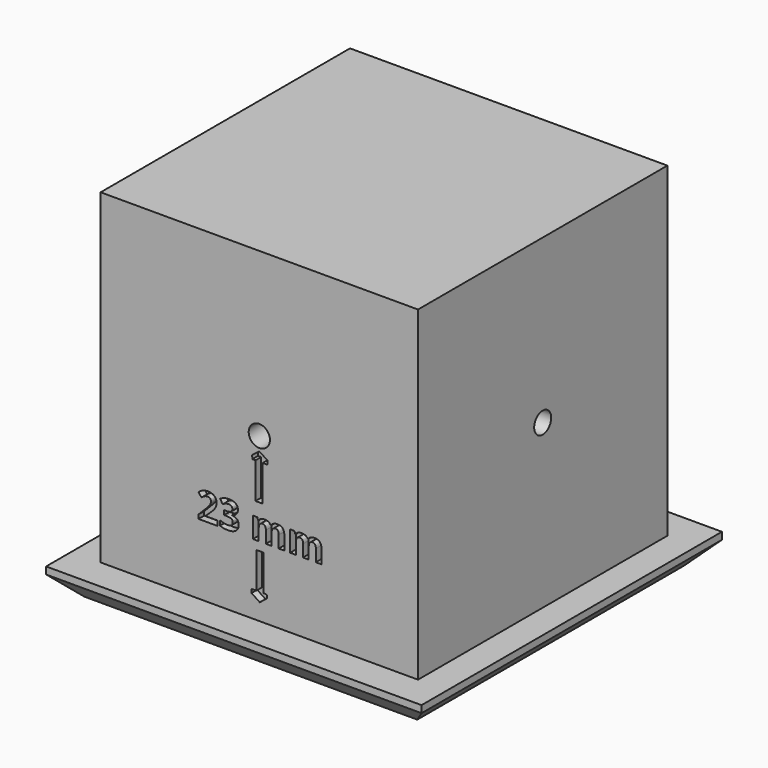
from build123d import *

# Parameters (mm, degrees)
F0_W          = 44.8
F0_H          = 44
F0_W_2        = 37.5
F0_H_2        = 37.5
F1_DEPTH      = 50
F2_DEPTH      = 45.6
F4_W          = 53
F4_H          = 53
F5_DEPTH      = 4
F6_SIZE       = 3
F7_R          = 1.5
F8_DEPTH      = 44.8
F9_R          = 1.5
F10_DEPTH     = 44
F11_TEXT_SIZE = 5.341881317
F12_DEPTH     = 1


# Not quite as in the source:
# - Text() gives the source's letters only with a copy of the font that has no kerning and outlines rounded to 1/6400 em; it was checked with that copy


with BuildPart() as f1:
    # F0 (on Top) → F1 (new body)
    with BuildSketch(Plane.XY):
        Rectangle(F0_W, F0_H)
        Rectangle(F0_W_2, F0_H_2, mode=Mode.SUBTRACT)
        Rectangle(F0_W_2, F0_H_2)
    extrude(amount=F1_DEPTH)

    # F0 (on Top) → F2 (cut)
    with BuildSketch(Plane.XY):
        Rectangle(F0_W_2, F0_H_2)
    extrude(amount=F2_DEPTH, mode=Mode.SUBTRACT)

    # F4 (on offset) → F5 (join, through all)
    with BuildSketch(Plane.XY.offset(4)):
        Rectangle(F4_W, F4_H)
        Polygon((21.5723104775, -21.085973829), (-21.0834983736, -20.8649747074), (-21.0834983736, 21.5922761708), (21.5723104775, 21.5922761708), align=None, mode=Mode.SUBTRACT)
    extrude(amount=-F5_DEPTH)

    # F6
    f6_edges = [f1.edges().sort_by_distance(p)[0] for p in [
        (0, 26.5, 0),
        (26.5, 0, 0),
        (-26.5, 0, 0),
        (0, -26.5, 0),
    ]]
    chamfer(f6_edges, length=F6_SIZE)

    # F7 (on face) → F8 (cut, through all)
    with BuildSketch(Plane.YZ.offset(22.4)):
        with Locations((0, 27)):
            Circle(F7_R)
    extrude(amount=-F8_DEPTH, mode=Mode.SUBTRACT)

    # F9 (on face) → F10 (cut, through all)
    with BuildSketch(Plane.XZ.offset(22)):
        with Locations((0, 27)):
            Circle(F9_R)
    extrude(amount=-F10_DEPTH, mode=Mode.SUBTRACT)

    # F11 (on face) → F12 (cut)
    with BuildSketch(Plane.XZ.offset(22)):
        with Locations((-8.7980786338, 13.8999996707)):
            Text('23 mm', F11_TEXT_SIZE, font='Open Sans', font_style=FontStyle.BOLD, text_align=(TextAlign.LEFT, TextAlign.BOTTOM))
        Polygon((0, 25.0964813182), (-1.0096158367, 24.3076924235), (-0.983382226, 23.7985346466), (-0.5386771518, 23.7985346466), (-0.5386771518, 18.7450703233), (0.4720157012, 18.7450703233), (0.4720157012, 23.7985346466), (1.1592871742, 23.7985346466), (1.1592871742, 24.3240948766), align=None)
        Polygon((0.0613228767, 6.3521818941), (1.0709387134, 7.1409707889), (1.0447051027, 7.6501285657), (0.6000000285, 7.6501285657), (0.6000000285, 12.703592889), (-0.4106928245, 12.703592889), (-0.4106928245, 7.6501285657), (-1.0979642975, 7.6501285657), (-1.0979642975, 7.1245683357), align=None)
    extrude(amount=-F12_DEPTH, mode=Mode.SUBTRACT)


solid = f1.part
